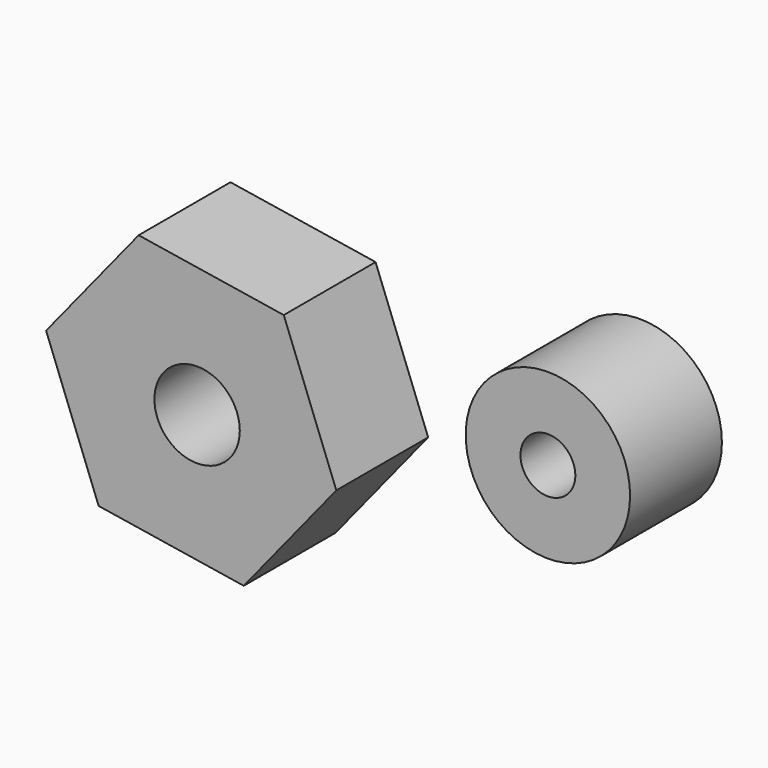
from build123d import *

# Parameters (mm, degrees)
F1_R      = 18.1896249191
F5_DEPTH  = 25.4
F6_R      = 6.0688570955
F7_DEPTH  = 27.2348383442
F9_DEPTH  = 25.4
F10_R     = 9.4468290058
F11_DEPTH = 25.4


# Not quite as in the source:
# - a feature of the source that left no trace in its solid (it failed there, or was rolled back) is left out


with BuildPart() as f5:
    # F1 (on Front) → F5 (new body)
    with BuildSketch(Plane.XZ):
        with Locations((46.8149334192, -8.7941288948)):
            Circle(F1_R)
    extrude(amount=F5_DEPTH)

    # F6 (on face) → F7 (cut)
    with BuildSketch(Plane(origin=(0, 0, 0), x_dir=(-1, 0, 0), z_dir=(0, 1, 0))):
        with Locations((-46.8149334192, -8.7941288948)):
            Circle(F6_R)
    extrude(amount=-F7_DEPTH, mode=Mode.SUBTRACT)


with BuildPart() as f9:
    # F8 (on Front) → F9 (new body)
    with BuildSketch(Plane.XZ):
        Polygon((-20.4813697214, -54.164792812), (0, -28.9118289948), (-11.6290233259, 1.4520393969), (-43.7394163733, 6.5629439713), (-64.2207860947, -18.690019846), (-52.5917627687, -49.0538882377), align=None)
    extrude(amount=F9_DEPTH)

    # F10 (on face) → F11 (cut)
    with BuildSketch(Plane.XZ.offset(25.4)):
        with Locations((-30.8052618057, -24.2253299803)):
            Circle(F10_R)
    extrude(amount=-F11_DEPTH, mode=Mode.SUBTRACT)


solid = Compound([f5.part, f9.part])
